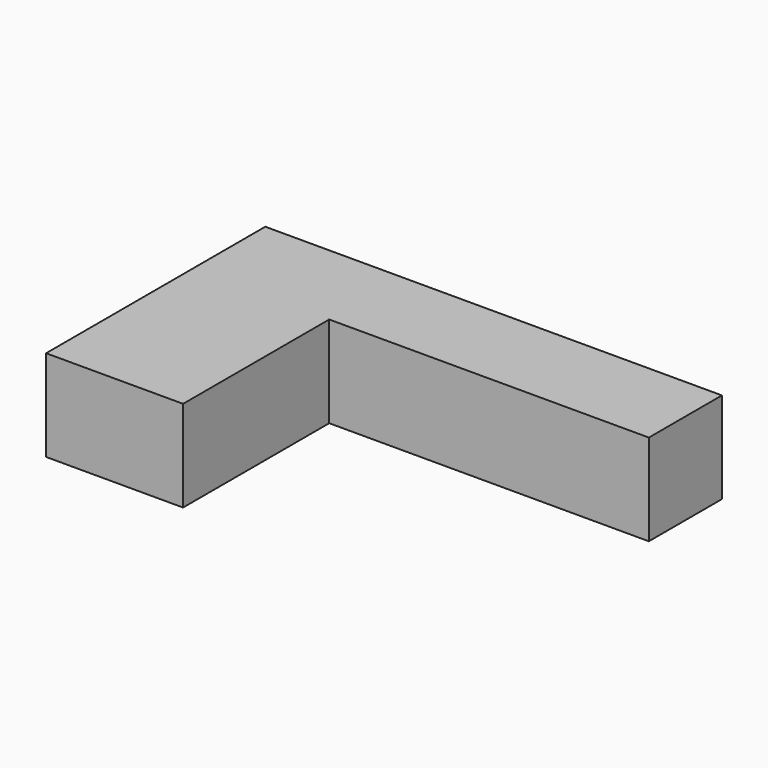
from build123d import *

# Parameters (mm, degrees)
F1_DEPTH = 12.7


# Not quite as in the source:
# - a length typed as a fraction of an inch, garbled in the dataset ("3 / 203.2 mm" for 3/8 in), is restored


with BuildPart() as f1:
    # F0 (on Top) → F1 (new body)
    with BuildSketch(Plane.XY):
        Polygon((-45.8524803743, 24.5433666376), (-45.8524803743, -13.5566333624), (-26.8024803743, -13.5566333624), (-26.8024803743, 11.8433666376), (17.6475196257, 11.8433666376), (17.6475196257, 24.5433666376), align=None)
    extrude(amount=F1_DEPTH)


solid = f1.part
